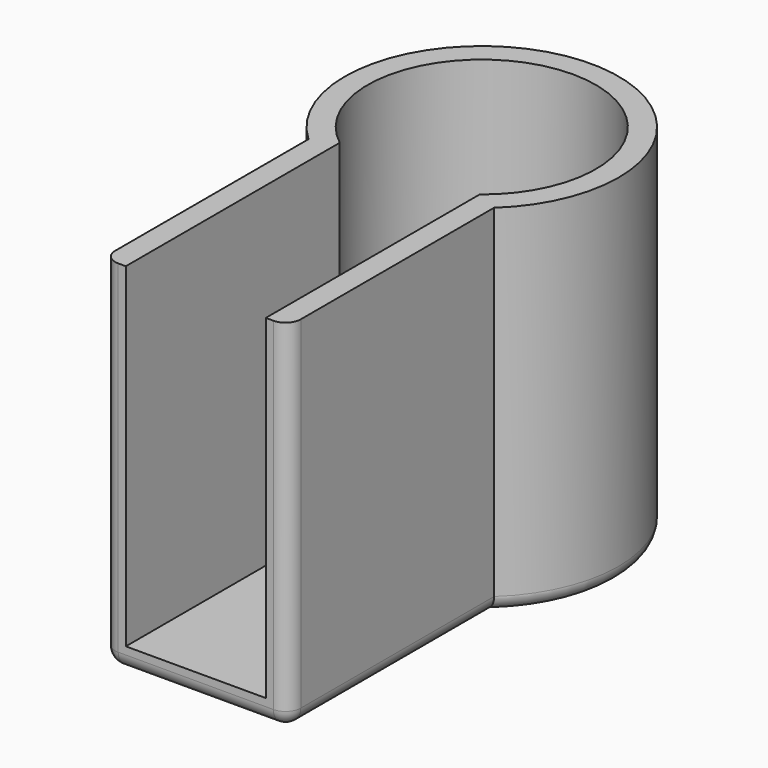
from build123d import *

# Parameters (mm, degrees)
F1_DEPTH = 22
F2_T     = 1.5
F3_W     = 9.2
F3_H     = 22
F4_DEPTH = 1.5
F5_R     = 1


with BuildPart() as f1:
    # F0 (on Top) → F1 (new body)
    with BuildSketch(Plane.XY):
        with BuildLine():
            Line((-4.6, -5.9236812878), (-4.6, -22))
            Line((-4.6, -22), (4.6, -22))
            Line((4.6, -22), (4.6, -5.9236812878))
            ThreePointArc((4.6, -5.9236812878), (0, 7.5), (-4.6, -5.9236812878))
        make_face()
    extrude(amount=F1_DEPTH)

    # F2
    f2_openings = [f1.faces().sort_by_distance(p)[0] for p in [
        (0, -6.355052, 22),
    ]]
    offset(amount=F2_T, openings=f2_openings, kind=Kind.INTERSECTION)

    # F3 (on face) → F4 (cut, through all)
    with BuildSketch(Plane.XZ.offset(23.5)):
        with Locations((0, 11)):
            Rectangle(F3_W, F3_H)
    extrude(amount=-F4_DEPTH, mode=Mode.SUBTRACT)

    # F5
    f5_edges = [f1.edges().sort_by_distance(p)[0] for p in [
        (6.1, -23.5, 10.25),
        (-6.1, -23.5, 10.25),
        (0, -23.5, -1.5),
        (-6.1, -15.058701, -1.5),
        (6.1, -15.058701, -1.5),
        (0, 9, -1.5),
    ]]
    fillet(f5_edges, radius=F5_R)


solid = f1.part
